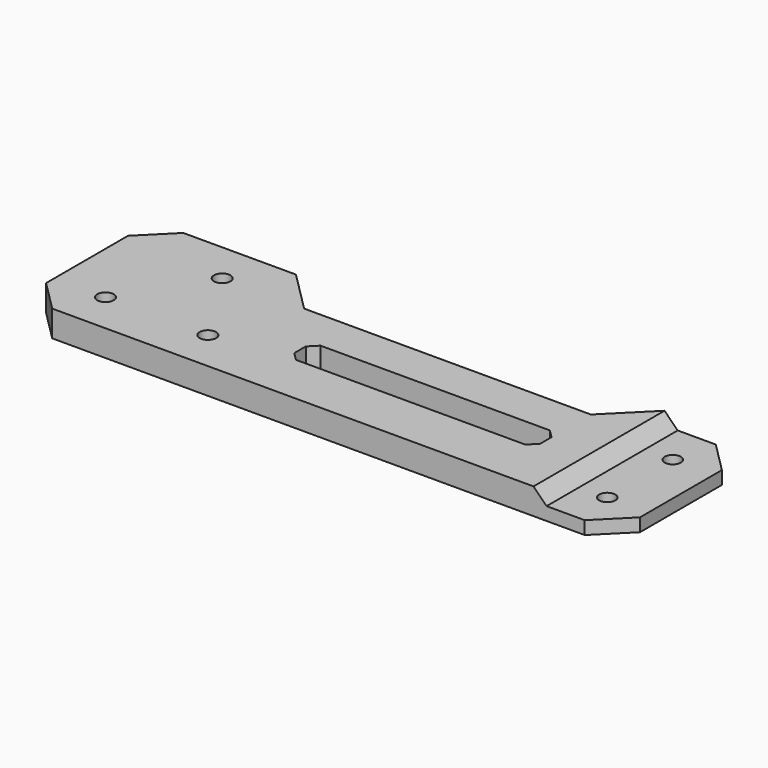
from build123d import *

# Parameters (mm, degrees)
F0_W      = 184.15
F0_H      = 50.8
F1_DEPTH  = 8.128
F3_D      = 5.1054
F6_D      = 4.9784
F7_W      = 76.2
F7_H      = 9.525
F8_DEPTH  = 8.129
F9_SIZE   = 9.525
F10_SIZE  = 2.54
F11_R     = 2.4892
F12_DEPTH = 4.064
F13_SIZE  = 4.06399


# Not quite as in the source:
# - a fillet or chamfer is up to 0.001 mm smaller than in the source, because OpenCascade refuses the exact size


with BuildPart() as f1:
    # F0 (on Top) → F1 (new body)
    with BuildSketch(Plane.XY):
        Rectangle(F0_W, F0_H)
    extrude(amount=F1_DEPTH)

    # F3 (through all)
    with Locations(Plane.XY.offset(8.128)):
        with Locations((-60.325, 12.7), (-76.2, -12.7), (-44.45, -12.7)):
            Hole(F3_D / 2)

    # F6 (through all)
    with Locations(Plane.XY.offset(8.128)):
        with Locations((79.375, 12.7), (79.375, -12.7)):
            Hole(F6_D / 2)

    # F7 (on face) → F8 (cut, through all)
    with BuildSketch(Plane.XY.offset(8.128)):
        Polygon((66.675, 25.4), (-47.625, 25.4), (-34.925, 12.7), (53.975, 12.7), align=None)
        with Locations((15.875, -4.7625)):
            Rectangle(F7_W, F7_H)
    extrude(amount=-F8_DEPTH, mode=Mode.SUBTRACT)

    # F9
    f9_edges = [f1.edges().sort_by_distance(p)[0] for p in [
        (-92.075, -25.4, 4.064),
        (-92.075, 25.4, 4.064),
        (92.075, -25.4, 4.064),
        (92.075, 25.4, 4.064),
    ]]
    chamfer(f9_edges, length=F9_SIZE)

    # F10
    f10_edges = [f1.edges().sort_by_distance(p)[0] for p in [
        (-22.225, 0, 4.064),
        (-22.225, -9.525, 4.064),
        (53.975, 0, 4.064),
        (53.975, -9.525, 4.064),
    ]]
    chamfer(f10_edges, length=F10_SIZE)

    # F11 (on face) → F12 (cut)
    with BuildSketch(Plane.XY.offset(8.128)):
        Polygon((82.55, 25.4), (66.675, 25.4), (66.675, -25.4), (82.55, -25.4), (92.075, -15.875), (92.075, 15.875), align=None)
        with Locations((79.375, -12.7)):
            Circle(F11_R, mode=Mode.SUBTRACT)
        with Locations((79.375, 12.7)):
            Circle(F11_R, mode=Mode.SUBTRACT)
    extrude(amount=-F12_DEPTH, mode=Mode.SUBTRACT)

    # F13 (size 4.064 in the source; OpenCascade refuses exactly that, so slightly less here)
    f13_edges = [f1.edges().sort_by_distance(p)[0] for p in [
        (66.675, 0, 4.064),
    ]]
    chamfer(f13_edges, length=F13_SIZE)


solid = f1.part
